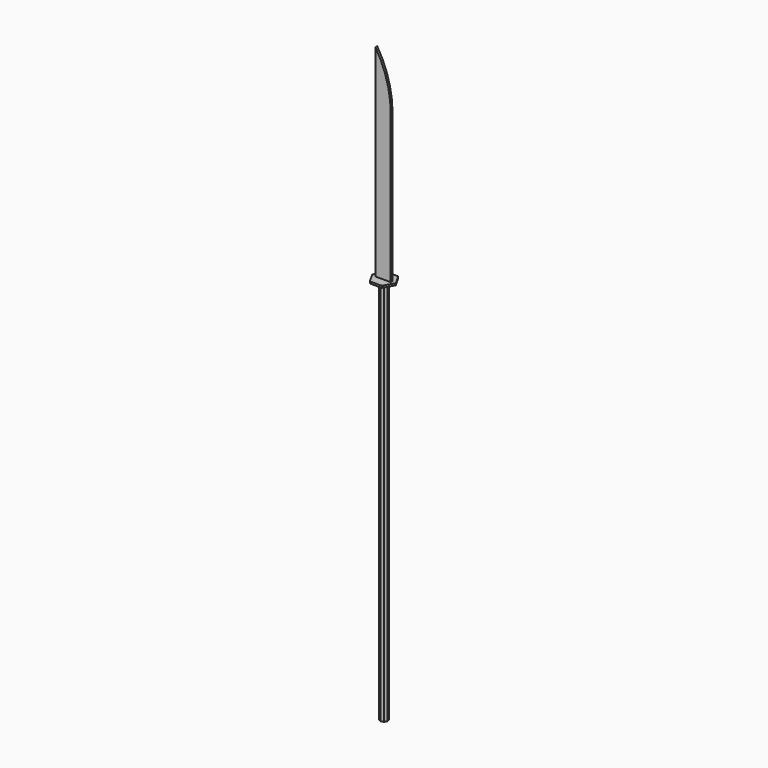
from build123d import *

# Parameters (mm, degrees)
F0_W        = 40.3080582619
F0_H        = 5.9715644456
F1_DEPTH    = 537
F3_DEPTH    = 1017
F5_DEPTH    = 5
F6_T1_DEPTH = 716.1336390313


# Not quite as in the source:
# - a fillet or chamfer that OpenCascade refuses, or shapes differently, is made with other operations: its cross-section is extruded or revolved along the edge and cut away or added


with BuildPart() as f1:
    # F0 (on Top) → F1 (new body)
    with BuildSketch(Plane.XY):
        Rectangle(F0_W, F0_H)
    extrude(amount=F1_DEPTH)

    # F2 (on Top) → F3 (join)
    with BuildSketch(Plane.XY):
        Polygon((6.5744029718, -8.407556447), (10.5938451005, -1.2962352533), (8.407556447, 6.5744029718), (1.2962352533, 10.5938451005), (-6.5744029718, 8.407556447), (-10.5938451005, 1.2962352533), (-8.407556447, -6.5744029718), (-1.2962352533, -10.5938451005), align=None)
    extrude(amount=-F3_DEPTH)

    # F4 (on Top) → F5 (join)
    with BuildSketch(Plane.XY):
        Polygon((31.1715127681, -0.1368859226), (15.7043030704, 26.9268789703), (-15.4672096977, 27.0637648929), (-31.1715127681, 0.1368859226), (-15.7043030704, -26.9268789703), (15.4672096977, -27.0637648929), align=None)
    extrude(amount=F5_DEPTH)

    # F6: fillet of radius 270.3919189858 on 1 edges, made by hand

    # F6_s2 → F6_t1 (cut)
    with BuildSketch(Plane.XZ.offset(-358.0668195157)):
        with BuildLine():
            ThreePointArc((-20.1540291309, 537), (9.881896476, 468.7882231999), (20.1540291309, 394.9675850829))
            Line((20.1540291309, 394.9675850829), (20.1540291309, 537))
            Line((20.1540291309, 537), (-20.1540291309, 537))
        make_face()
    extrude(amount=F6_T1_DEPTH, mode=Mode.SUBTRACT)


solid = f1.part
